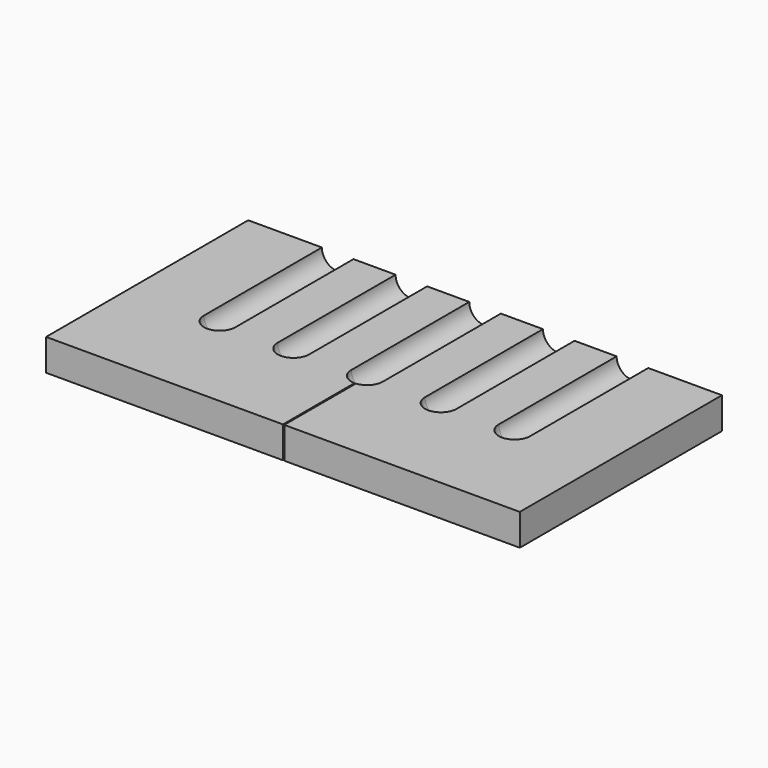
from build123d import *

# Parameters (mm, degrees)
F0_W     = 285.75
F0_H     = 152.4
F1_DEPTH = 19.05
F3_DEPTH = 9.525
F4_R     = 9.52499
F6_DEPTH = 25.4


# Not quite as in the source:
# - a fillet or chamfer is up to 0.001 mm smaller than in the source, because OpenCascade refuses the exact size


with BuildPart() as f1:
    # F0 (on Top) → F1 (new body)
    with BuildSketch(Plane.XY):
        with Locations((1.3537015766, -58.2166751785)):
            Rectangle(F0_W, F0_H)
    extrude(amount=F1_DEPTH)

    # F2 (on face) → F3 (cut)
    with BuildSketch(Plane.XY.offset(19.05)):
        with BuildLine():
            Line((-78.0212984234, 17.9833248215), (-97.0712984234, 17.9833248215))
            Line((-97.0712984234, 17.9833248215), (-97.0712984234, -70.9166751785))
            ThreePointArc((-97.0712984234, -70.9166751785), (-94.2814905142, -77.6518672693), (-87.5462984234, -80.4416751785))
            ThreePointArc((-87.5462984234, -80.4416751785), (-80.8111063326, -77.6518672693), (-78.0212984234, -70.9166751785))
            Line((-78.0212984234, -70.9166751785), (-78.0212984234, 17.9833248215))
        make_face()
        with BuildLine():
            Line((-33.5712984234, 17.9833248215), (-52.6212984234, 17.9833248215))
            Line((-52.6212984234, 17.9833248215), (-52.6212984234, -70.9166751785))
            ThreePointArc((-52.6212984234, -70.9166751785), (-49.8314905142, -77.6518672693), (-43.0962984234, -80.4416751785))
            ThreePointArc((-43.0962984234, -80.4416751785), (-36.3611063326, -77.6518672693), (-33.5712984234, -70.9166751785))
            Line((-33.5712984234, -70.9166751785), (-33.5712984234, 17.9833248215))
        make_face()
        with BuildLine():
            Line((10.8787015766, 17.9833248215), (-8.1712984234, 17.9833248215))
            Line((-8.1712984234, 17.9833248215), (-8.1712984234, -70.9166751785))
            ThreePointArc((-8.1712984234, -70.9166751785), (-5.3814905142, -77.6518672693), (1.3537015766, -80.4416751785))
            ThreePointArc((1.3537015766, -80.4416751785), (8.0888936674, -77.6518672693), (10.8787015766, -70.9166751785))
            Line((10.8787015766, -70.9166751785), (10.8787015766, 17.9833248215))
        make_face()
        with BuildLine():
            Line((55.3287015766, 17.9833248215), (36.2787015766, 17.9833248215))
            Line((36.2787015766, 17.9833248215), (36.2787015766, -70.9166751785))
            ThreePointArc((36.2787015766, -70.9166751785), (39.0685094858, -77.6518672693), (45.8037015766, -80.4416751785))
            ThreePointArc((45.8037015766, -80.4416751785), (52.5388936674, -77.6518672693), (55.3287015766, -70.9166751785))
            Line((55.3287015766, -70.9166751785), (55.3287015766, 17.9833248215))
        make_face()
        with BuildLine():
            Line((99.7787015766, -70.9166751785), (99.7787015766, 17.9833248215))
            Line((99.7787015766, 17.9833248215), (80.7287015766, 17.9833248215))
            Line((80.7287015766, 17.9833248215), (80.7287015766, -70.9166751785))
            ThreePointArc((80.7287015766, -70.9166751785), (83.5185094858, -77.6518672693), (90.2537015766, -80.4416751785))
            ThreePointArc((90.2537015766, -80.4416751785), (96.9888936674, -77.6518672693), (99.7787015766, -70.9166751785))
        make_face()
    extrude(amount=-F3_DEPTH, mode=Mode.SUBTRACT)

    # F4 (radius 9.525 in the source; OpenCascade refuses exactly that, so slightly less here)
    f4_edges = [f1.edges().sort_by_distance(p)[0] for p in [
        (-87.546298, -80.441675, 9.525),
        (-52.621298, -26.466675, 9.525),
        (-8.171298, -26.466675, 9.525),
        (36.278702, -26.466675, 9.525),
        (80.728702, -26.466675, 9.525),
    ]]
    fillet(f4_edges, radius=F4_R)

    # F5 (on face) → F6 (cut)
    with BuildSketch(Plane.XY.offset(19.05)):
        with BuildLine():
            Line((1.3537015766, 17.9833248215), (1.3537015766, -80.4416751785))
            ThreePointArc((1.3537015766, -80.4416751785), (1.7509221371, -80.4333889404), (2.1474515766, -80.4085446434))
            Line((2.1474515766, -80.4085446434), (2.1474515766, 17.9833248215))
            Line((2.1474515766, 17.9833248215), (1.3537015766, 17.9833248215))
        make_face()
        with BuildLine():
            Line((1.3537015766, -80.4416751785), (1.3537015766, -134.4166751785))
            Line((1.3537015766, -134.4166751785), (2.1474515766, -134.4166751785))
            Line((2.1474515766, -134.4166751785), (2.1474515766, -80.4085446434))
            ThreePointArc((2.1474515766, -80.4085446434), (1.7509221371, -80.4333889404), (1.3537015766, -80.4416751785))
        make_face()
    extrude(amount=-F6_DEPTH, mode=Mode.SUBTRACT)


solid = f1.part
